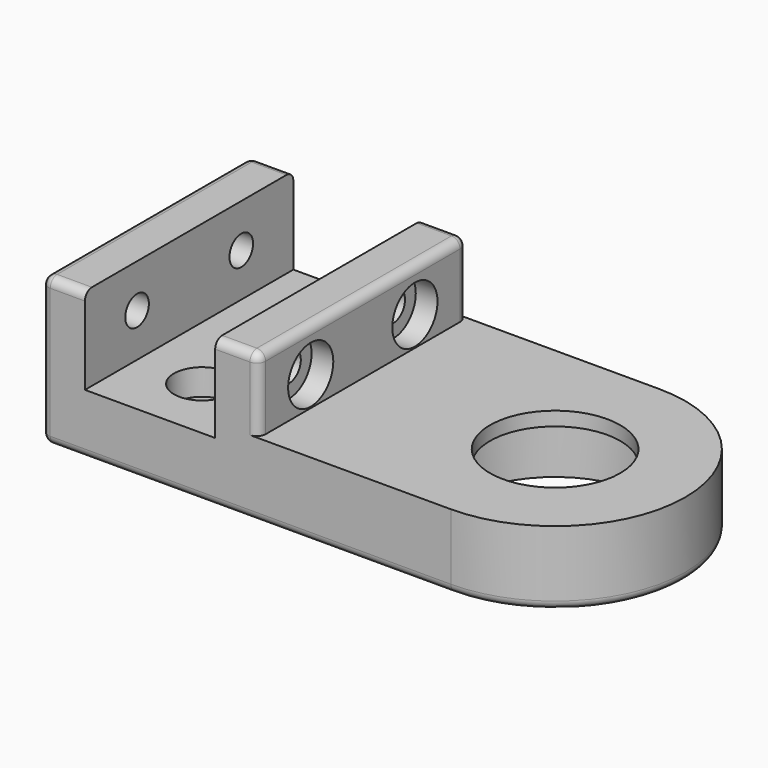
from build123d import *

# Parameters (mm, degrees)
F0_R          = 11.1
F1_DEPTH      = 7
F2_W          = 5
F2_H          = 30
F3_DEPTH      = 10
F4_R          = 1.7
F5_DEPTH      = 5.001
F6_R          = 3.25
F7_DEPTH      = 2.5
F8_R          = 1.7
F9_DEPTH      = 25.001
F10_R         = 3.25
F11_DEPTH     = 2.5
F12_R         = 7.5
F13_DEPTH     = 1.6
F14_R         = 1
F15_R         = 1.7
F16_DEPTH     = 7.001
F17_R         = 3.25
F18_DEPTH     = 3
F19_T1_DEPTH  = 6.5
F19_T3_DEPTH  = 6.5
F19_S7_W      = 1
F19_S7_H      = 1
F19_T8_DEPTH  = 1
F19_S13_W     = 1
F19_S13_H     = 1
F19_T14_DEPTH = 1
F19_S19_W     = 1
F19_S19_H     = 1
F19_T20_DEPTH = 1
F19_S25_W     = 1
F19_S25_H     = 1
F19_T26_DEPTH = 1


# Not quite as in the source:
# - a fillet or chamfer that OpenCascade refuses, or shapes differently, is made with other operations: its cross-section is extruded or revolved along the edge and cut away or added


with BuildPart() as f1:
    # F0 (on Top) → F1 (new body)
    with BuildSketch(Plane.XY):
        with BuildLine():
            Line((-47.15, -15), (0, -15))
            ThreePointArc((0, -15), (15, 0), (0, 15))
            Line((0, 15), (-47.15, 15))
            Line((-47.15, 15), (-47.15, -15))
        make_face()
        Circle(F0_R, mode=Mode.SUBTRACT)
    extrude(amount=F1_DEPTH)

    # F2 (on face) → F3 (join)
    with BuildSketch(Plane.XY.offset(7)):
        with Locations((-44.65, 0)):
            Rectangle(F2_W, F2_H)
        with Locations((-24.65, 0)):
            Rectangle(F2_W, F2_H)
    extrude(amount=F3_DEPTH)

    # F4 (on face) → F5 (cut, through all)
    with BuildSketch(Plane.YZ.offset(-42.15)):
        with Locations((7.5, 12)):
            Circle(F4_R)
        with Locations((-7.5, 12)):
            Circle(F4_R)
    extrude(amount=-F5_DEPTH, mode=Mode.SUBTRACT)

    # F6 (on face) → F7 (cut)
    with BuildSketch(Plane(origin=(-47.15, 0, 0), x_dir=(0, -1, 0), z_dir=(-1, 0, 0))):
        with Locations((-7.5, 12)):
            Circle(F6_R)
        with Locations((7.5, 12)):
            Circle(F6_R)
    extrude(amount=-F7_DEPTH, mode=Mode.SUBTRACT)

    # F8 (on face) → F9 (cut, through all)
    with BuildSketch(Plane.YZ.offset(-22.15)):
        with Locations((7.5, 12)):
            Circle(F8_R)
        with Locations((-7.5, 12)):
            Circle(F8_R)
    extrude(amount=-F9_DEPTH, mode=Mode.SUBTRACT)

    # F10 (on face) → F11 (cut)
    with BuildSketch(Plane.YZ.offset(-22.15)):
        with Locations((7.5, 12)):
            Circle(F10_R)
        with Locations((-7.5, 12)):
            Circle(F10_R)
    extrude(amount=-F11_DEPTH, mode=Mode.SUBTRACT)

    # F12 (on face) → F13 (join)
    with BuildSketch(Plane.XY.offset(7)):
        with BuildLine():
            ThreePointArc((0, -15), (15, 0), (0, 15))
            Line((0, 15), (-22.15, 15))
            Line((-22.15, 15), (-22.15, -15))
            Line((-22.15, -15), (0, -15))
        make_face()
        Circle(F12_R, mode=Mode.SUBTRACT)
    extrude(amount=F13_DEPTH)

    # F14
    f14_edges = [f1.edges().sort_by_distance(p)[0] for p in [
        (-47.15, 0, 0),
        (-23.575, -15, 0),
        (15, 0, 0),
        (-23.575, 15, 0),
        (-47.15, -15, 8.5),
        (-47.15, 15, 8.5),
        (-47.15, 0, 17),
        (-22.15, 0, 17),
        (-22.15, -15, 12.8),
        (-22.15, 15, 12.8),
    ]]
    fillet(f14_edges, radius=F14_R)

    # F15 (on face) → F16 (cut, through all)
    with BuildSketch(Plane.XY.offset(7)):
        with Locations((-34.65, -7.5)):
            Circle(F15_R)
        with Locations((-34.65, 7.5)):
            Circle(F15_R)
    extrude(amount=-F16_DEPTH, mode=Mode.SUBTRACT)

    # F17 (on face) → F18 (cut)
    with BuildSketch(Plane.XY.offset(7)):
        with Locations((-34.65, -7.5)):
            Circle(F17_R)
        with Locations((-34.65, 7.5)):
            Circle(F17_R)
    extrude(amount=-F18_DEPTH, mode=Mode.SUBTRACT)

    # F19: fillet of radius 1 on 4 edges, made by hand

    # F19_s2 → F19_t1 (cut)
    with BuildSketch(Plane.YZ.offset(-46.15)):
        with BuildLine():
            ThreePointArc((15, 16), (14.7071067812, 16.7071067812), (14, 17))
            Line((14, 17), (15, 17))
            Line((15, 17), (15, 16))
        make_face()
        with BuildLine():
            ThreePointArc((-14, 17), (-14.7071067812, 16.7071067812), (-15, 16))
            Line((-15, 16), (-15, 17))
            Line((-15, 17), (-14, 17))
        make_face()
    extrude(amount=F19_T1_DEPTH, mode=Mode.SUBTRACT)

    # F19_s4 → F19_t3 (cut)
    with BuildSketch(Plane.YZ.offset(-29.65)):
        with BuildLine():
            ThreePointArc((15, 16), (14.7071067812, 16.7071067812), (14, 17))
            Line((14, 17), (15, 17))
            Line((15, 17), (15, 16))
        make_face()
        with BuildLine():
            ThreePointArc((-14, 17), (-14.7071067812, 16.7071067812), (-15, 16))
            Line((-15, 16), (-15, 17))
            Line((-15, 17), (-14, 17))
        make_face()
    extrude(amount=F19_T3_DEPTH, mode=Mode.SUBTRACT)


with BuildPart() as f19_tool6:
    # F19_s7 → F19_t8 (new body)
    with BuildSketch(Plane.XY.offset(16)):
        with Locations((-46.65, -14.5)):
            Rectangle(F19_S7_W, F19_S7_H)
    extrude(amount=F19_T8_DEPTH)

    # F19_s9 → F19_t10 (revolve, cut)
    with BuildSketch(Plane(origin=(-46.15, -14, 16), x_dir=(0.7071067812, 0.7071067812, 0), z_dir=(0.7071067812, -0.7071067812, 0))):
        with BuildLine():
            ThreePointArc((0, -1), (1, 0), (0, 1))
            Line((0, 1), (0, -1))
        make_face()
    revolve(axis=Axis((-46.15, -14, 16), (0, 0, 1)), mode=Mode.SUBTRACT)


with BuildPart() as f1_1:
    add(f1.part)

    # F19_t5: cut F19_tool6
    add(f19_tool6.part, mode=Mode.SUBTRACT)


with BuildPart() as f19_tool12:
    # F19_s13 → F19_t14 (new body)
    with BuildSketch(Plane.XY.offset(16)):
        with Locations((-22.65, -14.5)):
            Rectangle(F19_S13_W, F19_S13_H)
    extrude(amount=F19_T14_DEPTH)

    # F19_s15 → F19_t16 (revolve, cut)
    with BuildSketch(Plane(origin=(-23.15, -14, 16), x_dir=(-0.7071067812, 0.7071067812, 0), z_dir=(0.7071067812, 0.7071067812, 0))):
        with BuildLine():
            ThreePointArc((0, -1), (1, 0), (0, 1))
            Line((0, 1), (0, -1))
        make_face()
    revolve(axis=Axis((-23.15, -14, 16), (0, 0, 1)), mode=Mode.SUBTRACT)


with BuildPart() as f1_2:
    add(f1_1.part)

    # F19_t11: cut F19_tool12
    add(f19_tool12.part, mode=Mode.SUBTRACT)


with BuildPart() as f19_tool18:
    # F19_s19 → F19_t20 (new body)
    with BuildSketch(Plane.XZ.offset(-14)):
        with Locations((-22.65, 16.5)):
            Rectangle(F19_S19_W, F19_S19_H)
    extrude(amount=-F19_T20_DEPTH)

    # F19_s21 → F19_t22 (revolve, cut)
    with BuildSketch(Plane(origin=(-23.15, 14, 16), x_dir=(-0.7071067812, 0, -0.7071067812), z_dir=(0.7071067812, 0, -0.7071067812))):
        with BuildLine():
            ThreePointArc((0, -1), (1, 0), (0, 1))
            Line((0, 1), (0, -1))
        make_face()
    revolve(axis=Axis((-23.15, 14, 16), (0, 1, 0)), mode=Mode.SUBTRACT)


with BuildPart() as f1_3:
    add(f1_2.part)

    # F19_t17: cut F19_tool18
    add(f19_tool18.part, mode=Mode.SUBTRACT)


with BuildPart() as f19_tool24:
    # F19_s25 → F19_t26 (new body)
    with BuildSketch(Plane.XZ.offset(-14)):
        with Locations((-46.65, 16.5)):
            Rectangle(F19_S25_W, F19_S25_H)
    extrude(amount=-F19_T26_DEPTH)

    # F19_s27 → F19_t28 (revolve, cut)
    with BuildSketch(Plane(origin=(-46.15, 14, 16), x_dir=(0.7071067812, 0, -0.7071067812), z_dir=(0.7071067812, 0, 0.7071067812))):
        with BuildLine():
            ThreePointArc((0, -1), (1, 0), (0, 1))
            Line((0, 1), (0, -1))
        make_face()
    revolve(axis=Axis((-46.15, 14, 16), (0, 1, 0)), mode=Mode.SUBTRACT)


with BuildPart() as f1_4:
    add(f1_3.part)

    # F19_t23: cut F19_tool24
    add(f19_tool24.part, mode=Mode.SUBTRACT)


solid = f1_4.part
